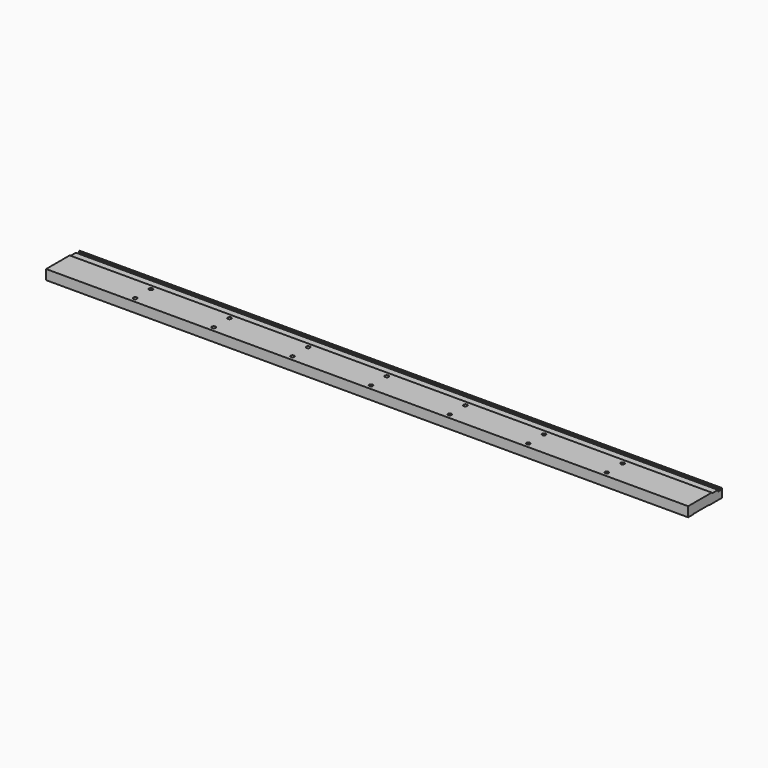
from build123d import *

# Parameters (mm, degrees)
F0_W           = 14.224
F0_H           = 20.574
F1_DEPTH       = 1244.6
F3_D           = 14.2875
F3_CBORE_D     = 21.43125
F3_CBORE_DEPTH = 13.49375
F4_SIZE        = 12.7


# Not quite as in the source:
# - a length typed as a fraction of an inch, garbled in the dataset ("3 / 203.2 mm" for 3/8 in), is restored


with BuildPart() as f1:
    # F0 (on Right) → F1 (new body, symmetric)
    with BuildSketch(Plane.YZ):
        Polygon((26.162, 19.05), (-88.138, 19.05), (-88.138, -19.05), (-62.738, -19.05), (-62.738, -17.526), (13.462, -17.526), (13.462, -19.05), (73.914, -19.05), (73.914, 1.524), (88.138, 1.524), (73.66, 16.002), (72.136, 16.002), (72.136, 9.652), (56.388, 9.652), (56.388, 16.002), (29.21, 16.002), align=None)
        with Locations((81.026, -8.763)):
            Rectangle(F0_W, F0_H)
    extrude(amount=F1_DEPTH, both=True)

    # F3 (through all)
    with Locations(Plane(origin=(0, 0, -19.05), x_dir=(1, 0, 0), z_dir=(0, 0, -1))):
        with Locations((914.4, -7.112), (914.4, 69.088), (609.6, 69.088), (609.6, -7.112), (304.8, -7.112), (304.8, 69.088), (0, -7.112), (0, 69.088), (-304.8, -7.112), (-304.8, 69.088), (-609.6, -7.112), (-609.6, 69.088), (-914.4, -7.112), (-914.4, 69.088)):
            CounterBoreHole(F3_D / 2, F3_CBORE_D / 2, F3_CBORE_DEPTH)

    # F4
    f4_edges = [f1.edges().sort_by_distance(p)[0] for p in [
        (1244.6, 88.138, -8.763),
        (-1244.6, 88.138, -8.763),
    ]]
    chamfer(f4_edges, length=F4_SIZE)


solid = f1.part
